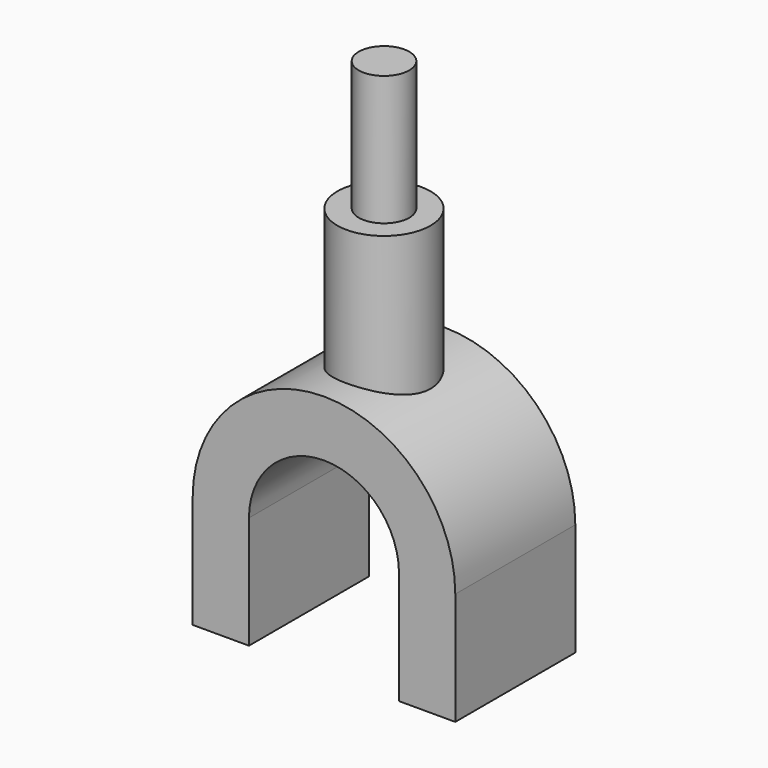
from build123d import *

# Parameters (mm, degrees)
F1_DEPTH = 25.4
F3_R     = 15.7727010677
F5_R     = 8.5503070877
F6_DEPTH = 43.942


with BuildPart() as f1:
    # F0 (on Front) → F1 (new body, symmetric)
    with BuildSketch(Plane.XZ):
        with BuildLine():
            ThreePointArc((-25.4, 0), (0, 25.4), (25.4, 0))
            Line((25.4, 0), (25.4, -38.1))
            Line((25.4, -38.1), (44.45, -38.1))
            Line((44.45, -38.1), (44.45, 0))
            ThreePointArc((44.45, 0), (0, 44.45), (-44.45, 0))
            Line((-44.45, 0), (-44.45, -38.1))
            Line((-44.45, -38.1), (-25.4, -38.1))
            Line((-25.4, -38.1), (-25.4, 0))
        make_face()
    extrude(amount=F1_DEPTH, both=True)

    # F3 (on offset) → F4 (join, up to the next surface of F1)
    with BuildSketch(Plane.XY.offset(90.17)):
        Circle(F3_R)
    extrude(until=Until.NEXT, dir=(0, 0, -1))

    # F5 (on offset) → F6 (join, symmetric)
    with BuildSketch(Plane.XY.offset(90.17)):
        Circle(F5_R)
    extrude(amount=F6_DEPTH, both=True)


solid = f1.part
